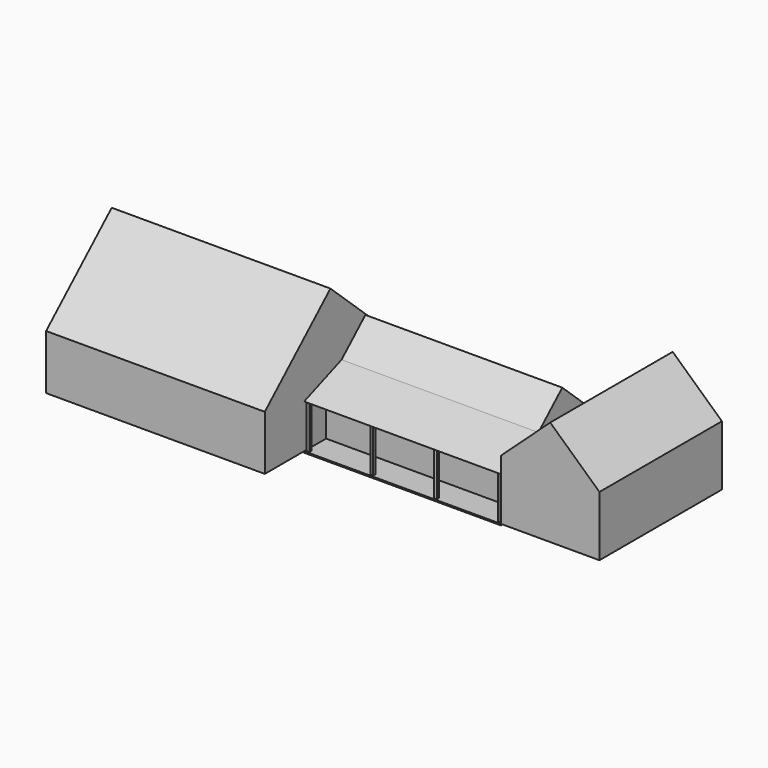
from build123d import *

# Parameters (mm, degrees)
F1_DEPTH  = 3048
F3_DEPTH  = 12192
F4_DEPTH  = 2438.4
F6_DEPTH  = 10972.8
F7_DEPTH  = 3352.8
F0_W      = 10972.8
F0_H      = 1524
F0_W_2    = 152.4
F0_H_2    = 152.4
F8_DEPTH  = 76.2
F9_DEPTH  = 2438.4
F11_DEPTH = 8534.4
F12_DEPTH = 2438.4
F13_DEPTH = 2438.4
F14_DEPTH = 2438.4


with BuildPart() as f1:
    # F0 (on Top) → F1 (new body)
    with BuildSketch(Plane.XY):
        Polygon((0, -1524), (0, 0), (0, 4876.8), (-12192, 4876.8), (-12192, -4267.2), (0, -4267.2), align=None)
    extrude(amount=F1_DEPTH)

    # F2 (on face) → F3 (join, through all)
    with BuildSketch(Plane(origin=(-12192, 0, 0), x_dir=(0, -1, 0), z_dir=(-1, 0, 0))):
        Polygon((4267.2, 3048), (-304.8, 7239), (-4876.8, 3048), align=None)
    extrude(amount=-F3_DEPTH)

    # F0 (on Top) → F4 (join)
    with BuildSketch(Plane.XY):
        Polygon((0, 4876.8), (0, 0), (10972.8, 0), (10972.8, 5486.4), (0, 5486.4), align=None)
    extrude(amount=F4_DEPTH)

    # F5 (on face) → F6 (join, through all)
    with BuildSketch(Plane.YZ.offset(10972.8)):
        Polygon((2743.2, 4953), (1081.5687689554, 3429.8380382092), (-1524, 2438.4), (0, 2438.4), (5486.4, 2438.4), align=None)
    extrude(amount=-F6_DEPTH)

    # F0 (on Top) → F7 (join)
    with BuildSketch(Plane.XY):
        Polygon((10972.8, 5486.4), (10972.8, 0), (10972.8, -1524), (16459.2, -1524), (16459.2, 7010.4), (10972.8, 7010.4), align=None)
    extrude(amount=F7_DEPTH)



with BuildPart() as f8:
    # F0 (on Top) → F8 (new body)
    with BuildSketch(Plane.XY):
        with Locations((5486.4, -762)):
            Rectangle(F0_W, F0_H)
        with Locations((152.4, -1371.6)):
            Rectangle(F0_W_2, F0_H_2, mode=Mode.SUBTRACT)
        with Locations((3708.4, -1371.6)):
            Rectangle(F0_W_2, F0_H_2, mode=Mode.SUBTRACT)
        with Locations((7264.4, -1371.6)):
            Rectangle(F0_W_2, F0_H_2, mode=Mode.SUBTRACT)
        with Locations((10820.4, -1371.6)):
            Rectangle(F0_W_2, F0_H_2, mode=Mode.SUBTRACT)
    extrude(amount=-F8_DEPTH)


with BuildPart() as f1_1:
    add(f1.part)

    add(f8.part)  # F9 merges F8
    # F0 (on Top) → F9 (join, through all)
    with BuildSketch(Plane.XY):
        with Locations((152.4, -1371.6)):
            Rectangle(F0_W_2, F0_H_2)
    extrude(amount=F9_DEPTH)

    # F10 (on face) → F11 (join, through all)
    with BuildSketch(Plane.XZ.offset(1524)):
        Polygon((13716, 5867.4), (10972.8, 3352.8), (16459.2, 3352.8), align=None)
    extrude(amount=-F11_DEPTH)

    # F0 (on Top) → F12 (join, through all)
    with BuildSketch(Plane.XY):
        with Locations((10820.4, -1371.6)):
            Rectangle(F0_W_2, F0_H_2)
    extrude(amount=F12_DEPTH)

    # F0 (on Top) → F13 (join, through all)
    with BuildSketch(Plane.XY):
        with Locations((7264.4, -1371.6)):
            Rectangle(F0_W_2, F0_H_2)
    extrude(amount=F13_DEPTH)

    # F0 (on Top) → F14 (join, through all)
    with BuildSketch(Plane.XY):
        with Locations((3708.4, -1371.6)):
            Rectangle(F0_W_2, F0_H_2)
    extrude(amount=F14_DEPTH)


solid = f1_1.part
